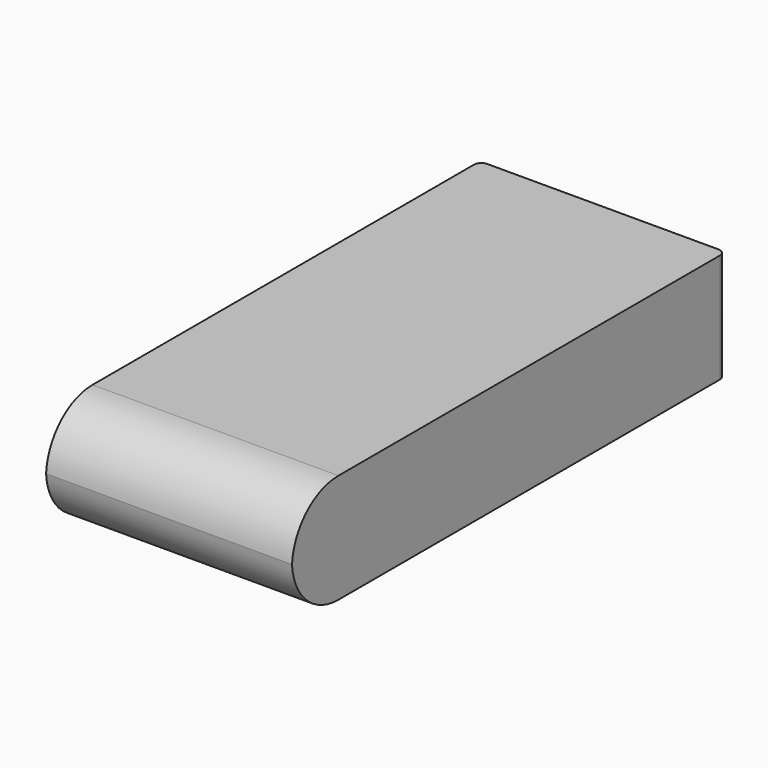
from build123d import *

# Parameters (mm, degrees)
F0_W        = 32.8
F0_H        = 14.57
F1_DEPTH    = 72.34
F2_T1_DEPTH = 71.55
F3_R        = 1


# Not quite as in the source:
# - a fillet or chamfer that OpenCascade refuses, or shapes differently, is made with other operations: its cross-section is extruded or revolved along the edge and cut away or added


with BuildPart() as f1:
    # F0 (on Front) → F1 (new body)
    with BuildSketch(Plane.XZ):
        with Locations((16.4, 7.285)):
            Rectangle(F0_W, F0_H)
    extrude(amount=F1_DEPTH)

    # F2: fillet of radius 7.75 on 2 edges, made by hand

    # F2_s2 → F2_t1 (cut)
    with BuildSketch(Plane.YZ.offset(-19.375)):
        with BuildLine():
            ThreePointArc((-64.59, 14.57), (-70.0700775542, 12.3000775542), (-72.34, 6.82))
            Line((-72.34, 6.82), (-72.34, 14.57))
            Line((-72.34, 14.57), (-64.59, 14.57))
        make_face()
        with BuildLine():
            ThreePointArc((-64.59, 0), (-70.0700775542, 2.2699224458), (-72.34, 7.75))
            Line((-72.34, 7.75), (-72.34, 0))
            Line((-72.34, 0), (-64.59, 0))
        make_face()
    extrude(amount=F2_T1_DEPTH, mode=Mode.SUBTRACT)

    # F3
    f3_edges = [f1.edges().sort_by_distance(p)[0] for p in [
        (0, 0, 7.285),
        (32.8, 0, 7.285),
    ]]
    fillet(f3_edges, radius=F3_R)


solid = f1.part
